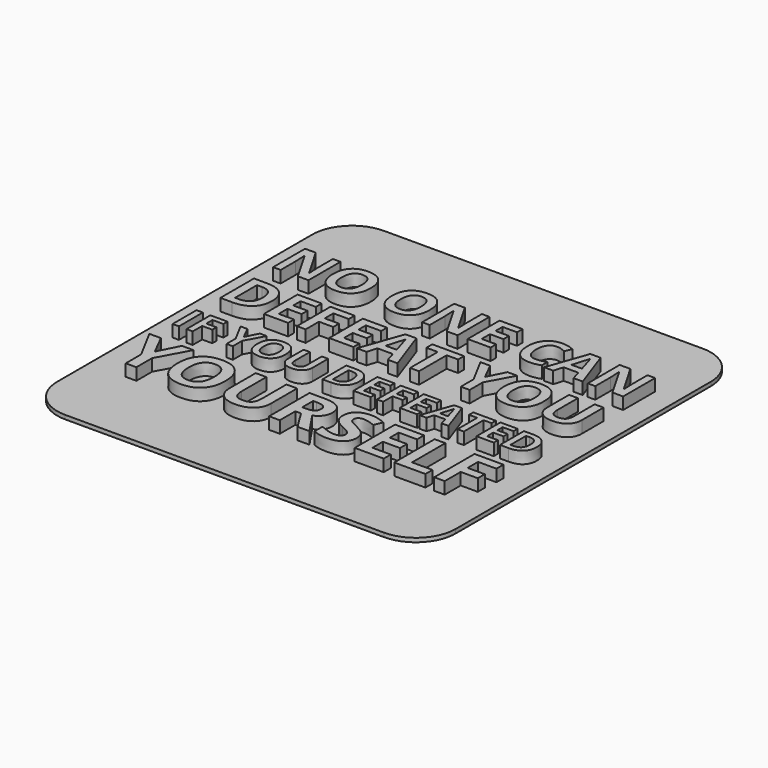
from build123d import *

# Parameters (mm, degrees)
F0_W           = 100
F0_H           = 100
F1_DEPTH       = 1
F2_TEXT_SIZE   = 14.0347457421
F2_TEXT_SIZE_2 = 14.7688520807
F2_TEXT_SIZE_3 = 10.5128673116
F2_TEXT_SIZE_4 = 17.7312605818
F3_DEPTH       = 3
F4_R           = 10


# Not quite as in the source:
# - Text() gives the source's letters only with a copy of the font that has no kerning and outlines rounded to 1/6400 em; it was checked with that copy


with BuildPart() as f1:
    # F0 (on Top) → F1 (new body)
    with BuildSketch(Plane.XY):
        Rectangle(F0_W, F0_H)
    extrude(amount=F1_DEPTH)

    # F2 (on face) → F3 (join)
    with BuildSketch(Plane.XY.offset(1)):
        with Locations((-45, 19.8949830657)):
            Text('NO ONE CAN', F2_TEXT_SIZE, font='Open Sans', font_style=FontStyle.BOLD, text_align=(TextAlign.LEFT, TextAlign.BOTTOM))
        with Locations((-45, 3.2614095676)):
            Text('DEFEAT YOU', F2_TEXT_SIZE_2, font='Open Sans', font_style=FontStyle.BOLD, text_align=(TextAlign.LEFT, TextAlign.BOTTOM))
        with Locations((-45, -11.2334923811)):
            Text('IF YOU DEFEATED', F2_TEXT_SIZE_3, font='Open Sans', font_style=FontStyle.BOLD, text_align=(TextAlign.LEFT, TextAlign.BOTTOM))
        with Locations((-45, -30)):
            Text('YOURSELF', F2_TEXT_SIZE_4, font='Open Sans', font_style=FontStyle.BOLD, text_align=(TextAlign.LEFT, TextAlign.BOTTOM))
    extrude(amount=F3_DEPTH)

    # F4
    f4_edges = [f1.edges().sort_by_distance(p)[0] for p in [
        (-50, 50, 0.5),
        (50, 50, 0.5),
        (-50, -50, 0.5),
        (50, -50, 0.5),
    ]]
    fillet(f4_edges, radius=F4_R)


solid = f1.part
